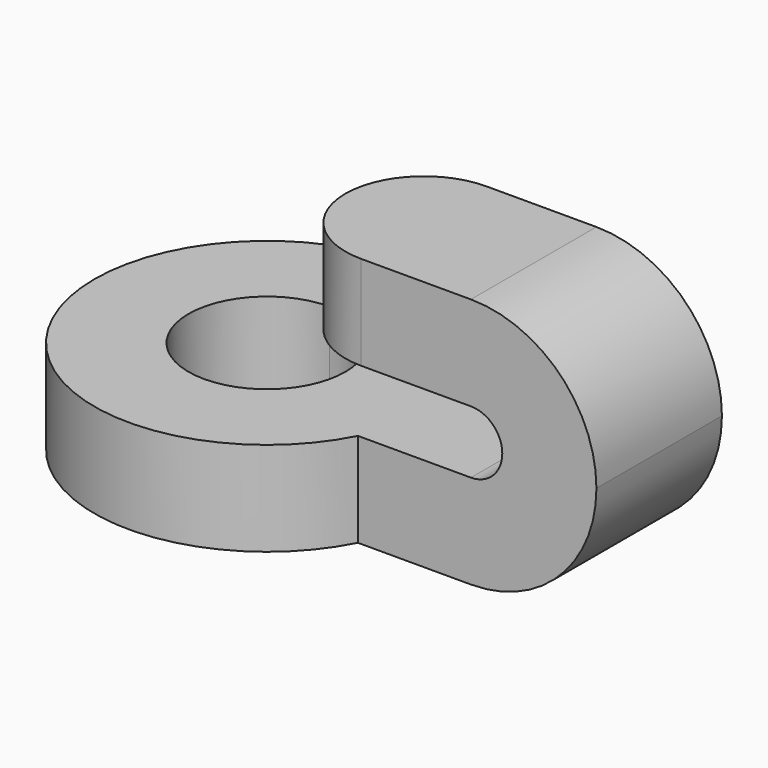
from build123d import *

# Parameters (mm, degrees)
F1_DEPTH = 3
F3_DEPTH = 5
F4_R     = 2.49999


# Not quite as in the source:
# - a fillet or chamfer is up to 0.001 mm smaller than in the source, because OpenCascade refuses the exact size


with BuildPart() as f1:
    # F0 (on Top) → F1 (new body)
    with BuildSketch(Plane.XY):
        with BuildLine():
            ThreePointArc((0, 2.5), (1.767766953, 1.767766953), (2.5, 0))
            ThreePointArc((2.5, 0), (1.767766953, -1.767766953), (0, -2.5))
            Line((0, -2.5), (4.8989794856, -2.5))
            ThreePointArc((4.8989794856, -2.5), (5.3476343915, -1.2856151892), (5.5, 0))
            ThreePointArc((5.5, 0), (5.3476343915, 1.2856151892), (4.8989794856, 2.5))
            Line((4.8989794856, 2.5), (0, 2.5))
        make_face()
        with BuildLine():
            ThreePointArc((0, -2.5), (-2.5, 0), (0, 2.5))
            Line((0, 2.5), (4.8989794856, 2.5))
            ThreePointArc((4.8989794856, 2.5), (-5.5, 0), (4.8989794856, -2.5))
            Line((4.8989794856, -2.5), (0, -2.5))
        make_face()
        with BuildLine():
            Line((8.5, 2.5), (4.8989794856, 2.5))
            ThreePointArc((4.8989794856, 2.5), (5.3476343915, 1.2856151892), (5.5, 0))
            ThreePointArc((5.5, 0), (5.3476343915, -1.2856151892), (4.8989794856, -2.5))
            Line((4.8989794856, -2.5), (8.5, -2.5))
            Line((8.5, -2.5), (8.5, 2.5))
        make_face()
    extrude(amount=F1_DEPTH)

    # F2 (on face) → F3 (join, through all)
    with BuildSketch(Plane.XZ.offset(2.5)):
        with BuildLine():
            Line((2.5, 5), (4.6270166538, 5))
            ThreePointArc((4.6270166538, 5), (6.0505102572, 7.1622776602), (8.5, 8))
            Line((8.5, 8), (2.5, 8))
            Line((2.5, 8), (2.5, 5))
        make_face()
        with BuildLine():
            Line((8.5, 0), (8.5, 3))
            Line((8.5, 3), (4.8989794856, 3))
            Line((4.8989794856, 3), (4.8989794856, 2.258549095))
            ThreePointArc((4.8989794856, 2.258549095), (6.3746533953, 0.6113569368), (8.5, 0))
        make_face()
        with BuildLine():
            ThreePointArc((8.5, 5), (9.2071067812, 4.7071067812), (9.5, 4))
            ThreePointArc((9.5, 4), (9.2071067812, 3.2928932188), (8.5, 3))
            Line((8.5, 3), (8.5, 0))
            ThreePointArc((8.5, 0), (11.3284271247, 1.1715728753), (12.5, 4))
            ThreePointArc((12.5, 4), (11.3284271247, 6.8284271247), (8.5, 8))
            ThreePointArc((8.5, 8), (6.0505102572, 7.1622776602), (4.6270166538, 5))
            Line((4.6270166538, 5), (8.5, 5))
        make_face()
    extrude(amount=-F3_DEPTH)

    # F4 (radius 2.5 in the source; OpenCascade refuses exactly that, so slightly less here)
    f4_edges = [f1.edges().sort_by_distance(p)[0] for p in [
        (2.5, -2.5, 6.5),
        (2.5, 2.5, 6.5),
    ]]
    fillet(f4_edges, radius=F4_R)


solid = f1.part
